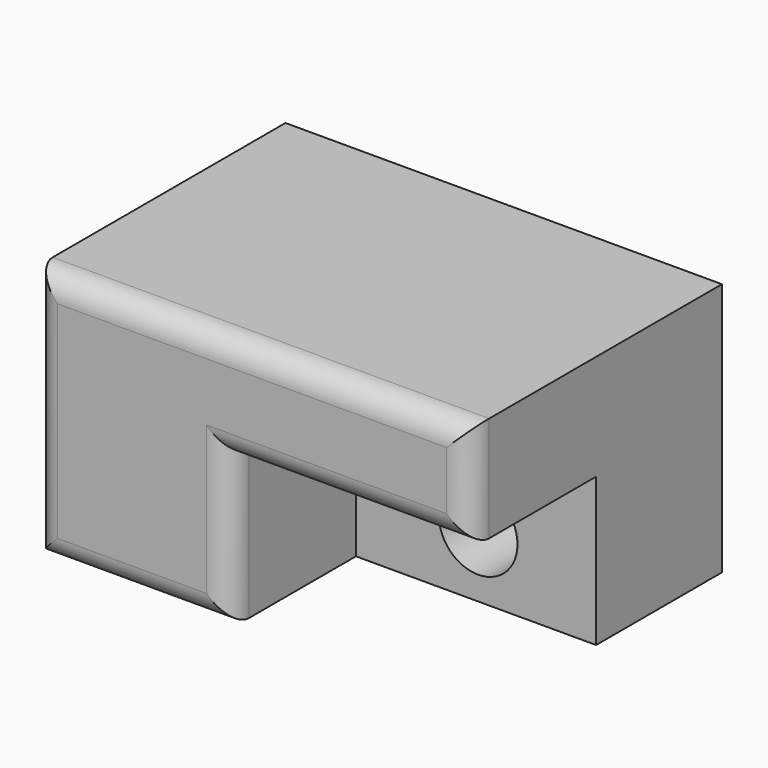
from build123d import *

# Parameters (mm, degrees)
F0_W     = 55.5101186037
F0_H     = 32.2702378035
F1_DEPTH = 40
F2_W     = 30.5438451469
F2_H     = 18.8575051725
F3_DEPTH = 20
F4_R     = 5
F5_DEPTH = 20.001
F7_R     = 3


# Not quite as in the source:
# - a feature of the source that left no trace in its solid (it failed there, or was rolled back) is left out


with BuildPart() as f1:
    # F0 (on Front) → F1 (new body)
    with BuildSketch(Plane.XZ):
        with Locations((27.7550593019, -16.1351189017)):
            Rectangle(F0_W, F0_H)
    extrude(amount=F1_DEPTH)

    # F2 (on face) → F3 (cut)
    with BuildSketch(Plane.XZ.offset(40)):
        with Locations((40.2381960303, -22.8414852172)):
            Rectangle(F2_W, F2_H)
    extrude(amount=-F3_DEPTH, mode=Mode.SUBTRACT)

    # F4 (on face) → F5 (cut, through all)
    with BuildSketch(Plane.XZ.offset(20)):
        with Locations((40.5101186037, -24.2702378035)):
            Circle(F4_R)
    extrude(amount=-F5_DEPTH, mode=Mode.SUBTRACT)

    # F7
    f7_edges = [f1.edges().sort_by_distance(p)[0] for p in [
        (24.966273, -40, -22.841485),
        (0, -40, -16.135119),
        (12.483137, -40, -32.270238),
        (40.238196, -40, -13.412733),
        (55.510119, -40, -6.706366),
        (27.755059, -40, 0),
    ]]
    fillet(f7_edges, radius=F7_R)


solid = f1.part
